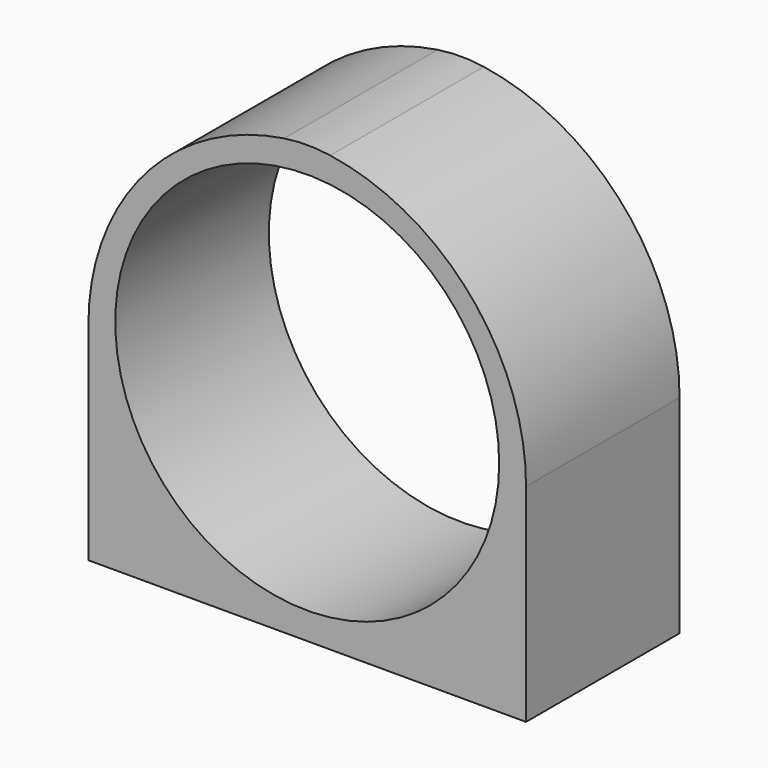
from build123d import *

# Parameters (mm, degrees)
F0_W        = 57
F0_H        = 57
F0_R        = 25
F1_DEPTH    = 25
F2_T1_DEPTH = 175
F3_R        = 20


# Not quite as in the source:
# - a fillet or chamfer that OpenCascade refuses, or shapes differently, is made with other operations: its cross-section is extruded or revolved along the edge and cut away or added


with BuildPart() as f1:
    # F0 (on Front) → F1 (new body)
    with BuildSketch(Plane.XZ):
        Rectangle(F0_W, F0_H)
        Circle(F0_R, mode=Mode.SUBTRACT)
    extrude(amount=F1_DEPTH)

    # F2: fillet of radius 30 on 2 edges, made by hand

    # F2_s2 → F2_t1 (cut)
    with BuildSketch(Plane.XZ.offset(-75)):
        with BuildLine():
            ThreePointArc((28.5, -1.5), (19.7132034356, 19.7132034356), (-1.5, 28.5))
            Line((-1.5, 28.5), (28.5, 28.5))
            Line((28.5, 28.5), (28.5, -1.5))
        make_face()
        with BuildLine():
            ThreePointArc((1.5, 28.5), (-19.7132034356, 19.7132034356), (-28.5, -1.5))
            Line((-28.5, -1.5), (-28.5, 28.5))
            Line((-28.5, 28.5), (1.5, 28.5))
        make_face()
    extrude(amount=F2_T1_DEPTH, mode=Mode.SUBTRACT)

    # F3
    f3_edges = [f1.edges().sort_by_distance(p)[0] for p in [
        (0, -12.5, 28.462477),
    ]]
    fillet(f3_edges, radius=F3_R)


solid = f1.part
